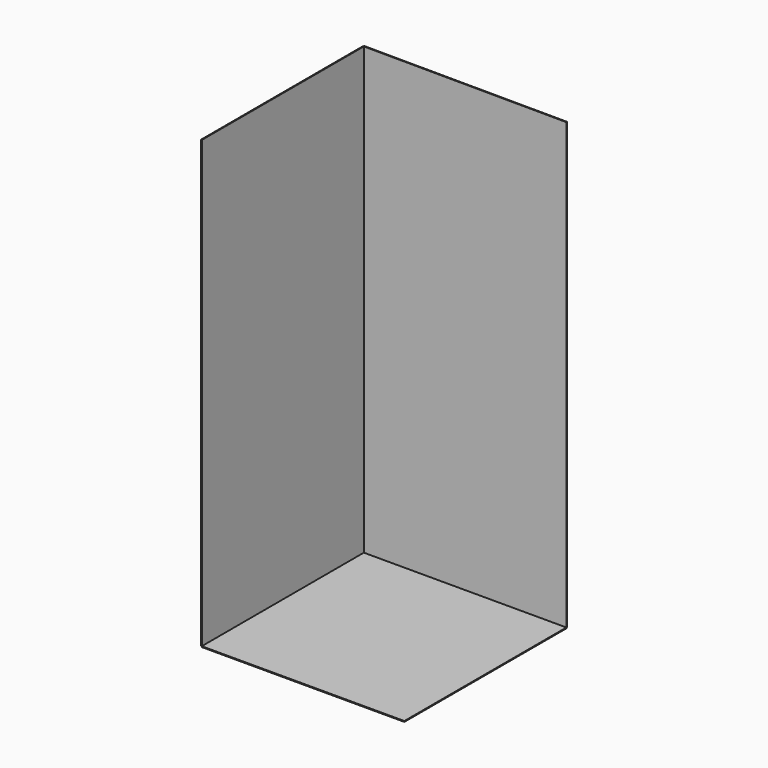
from build123d import *

# Parameters (mm, degrees)
F0_W     = 2540
F0_H     = 2540
F1_DEPTH = 10
F2_W     = 2540
F2_H     = 5588
F3_DEPTH = 10
F5_DEPTH = 10


# Not quite as in the source:
# - ends of sketch curves that miss each other by under 0.0002 mm in the source are joined


with BuildPart() as f1:
    # F0 (on Top) → F1 (new body)
    with BuildSketch(Plane.XY):
        with Locations((1270, 1270)):
            Rectangle(F0_W, F0_H)
    extrude(amount=F1_DEPTH)


with BuildPart() as f3:
    # F2 (on face) → F3 (new body)
    with BuildSketch(Plane(origin=(0, 0, 0), x_dir=(0, -1, 0), z_dir=(-1, 0, 0))):
        with Locations((-1270, 2804)):
            Rectangle(F2_W, F2_H)
    extrude(amount=F3_DEPTH)


with BuildPart() as f5:
    # F4 (on face) → F5 (new body)
    with BuildSketch(Plane(origin=(0, 2540, 0), x_dir=(-1, 0, 0), z_dir=(0, 1, 0))):
        Polygon((-2540, 10), (0, 10), (0, 5598), (-2539.9803148842, 5587.9999999653), align=None)
    extrude(amount=F5_DEPTH)


solid = Compound([f1.part, f3.part, f5.part])
